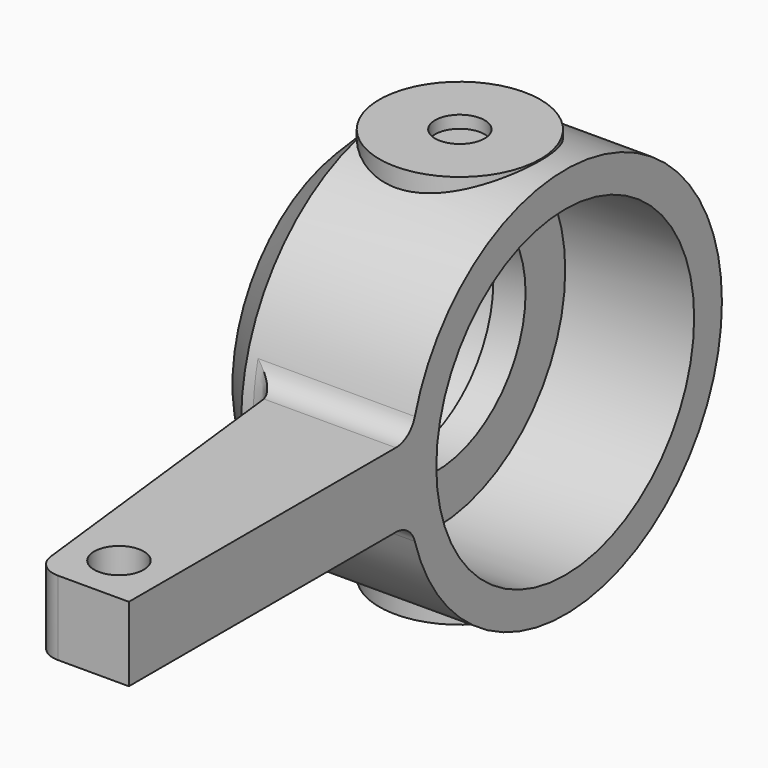
from build123d import *

# Parameters (mm, degrees)
F0_R         = 7.9
F1_DEPTH     = 4.25
F2_R         = 3.25
F3_DEPTH     = 7.95
F4_R         = 6.5
F5_DEPTH     = 5.2
F6_R         = 5.5
F7_DEPTH     = 2
F8_R         = 4.5
F9_DEPTH     = 8.5010001
F10_S5_R     = 3.25
F10_T6_DEPTH = 13
F12_DEPTH    = 1.5
F13_R        = 1
F14_R        = 1
F15_DEPTH    = 0.5
F16_R        = 1
F17_DEPTH    = 4
F18_R        = 1


# Not quite as in the source:
# - a fillet or chamfer that OpenCascade refuses, or shapes differently, is made with other operations: its cross-section is extruded or revolved along the edge and cut away or added
# - a pattern or mirror of a feature is missing from the dataset's text; its kind, count and spacing are read off the source's solid


with BuildPart() as f1:
    # F0 (on Right) → F1 (new body, symmetric)
    with BuildSketch(Plane.YZ):
        Circle(F0_R)
    extrude(amount=F1_DEPTH, both=True)

    # F2 (on Top) → F3 (join, symmetric)
    with BuildSketch(Plane.XY):
        Circle(F2_R)
    extrude(amount=F3_DEPTH, both=True)

    # F4 (on face) → F5 (cut)
    with BuildSketch(Plane.YZ.offset(4.25)):
        Circle(F4_R)
    extrude(amount=-F5_DEPTH, mode=Mode.SUBTRACT)

    # F6 (on face) → F7 (cut)
    with BuildSketch(Plane(origin=(-4.25, 0, 0), x_dir=(0, -1, 0), z_dir=(-1, 0, 0))):
        Circle(F6_R)
    extrude(amount=-F7_DEPTH, mode=Mode.SUBTRACT)

    # F8 (on face) → F9 (cut, through all)
    with BuildSketch(Plane.YZ.offset(4.25)):
        Circle(F8_R)
    extrude(amount=-F9_DEPTH, mode=Mode.SUBTRACT)

    # F10: chamfer of 1.75 on 1 edges, made by hand


with BuildPart() as f10_tool2:
    # F10_s3 → F10_t4 (revolve)
    with BuildSketch(Plane.XY):
        Polygon((-2.5, 7.9), (-4.25, 6.15), (-4.25, 7.9), align=None)
    revolve(axis=Axis((-4.25, 0, 0), (1, 0, 0)))

    # F10_s5 → F10_t6 (cut, symmetric)
    with BuildSketch(Plane.XY):
        Circle(F10_S5_R)
    extrude(amount=F10_T6_DEPTH, both=True, mode=Mode.SUBTRACT)


with BuildPart() as f1_1:
    add(f1.part)

    # F10_t1: cut F10_tool2
    add(f10_tool2.part, mode=Mode.SUBTRACT)

    # F11 (on Top) → F12 (join, symmetric)
    with BuildSketch(Plane.XY):
        Polygon((-1.25, -7), (0.5, -22), (4.25, -22), (4.25, -7), align=None)
    extrude(amount=F12_DEPTH, both=True)

    # F13
    f13_edges = [f1_1.edges().sort_by_distance(p)[0] for p in [
        (-1.145, -7.9, 0),
        (1.544117, -7.756288, 1.5),
        (1.544117, -7.756288, -1.5),
    ]]
    fillet(f13_edges, radius=F13_R)

    # F14 (on face) → F15 (cut)
    with BuildSketch(Plane.XY.offset(7.95)):
        Circle(F14_R)
    f15 = extrude(amount=-F15_DEPTH, mode=Mode.SUBTRACT)

    # F15_copies: F15 across plane
    add(f15.mirror(Plane(origin=(0, 0, 0), x_dir=(-1, 0, 0), z_dir=(0, 0, -1))), mode=Mode.SUBTRACT)

    # F16 (on Top) → F17 (cut, symmetric)
    with BuildSketch(Plane.XY):
        with Locations((2.25, -20)):
            Circle(F16_R)
    extrude(amount=F17_DEPTH, both=True, mode=Mode.SUBTRACT)

    # F18
    f18_edges = [f1_1.edges().sort_by_distance(p)[0] for p in [
        (0.5, -22, 0),
    ]]
    fillet(f18_edges, radius=F18_R)


solid = f1_1.part
